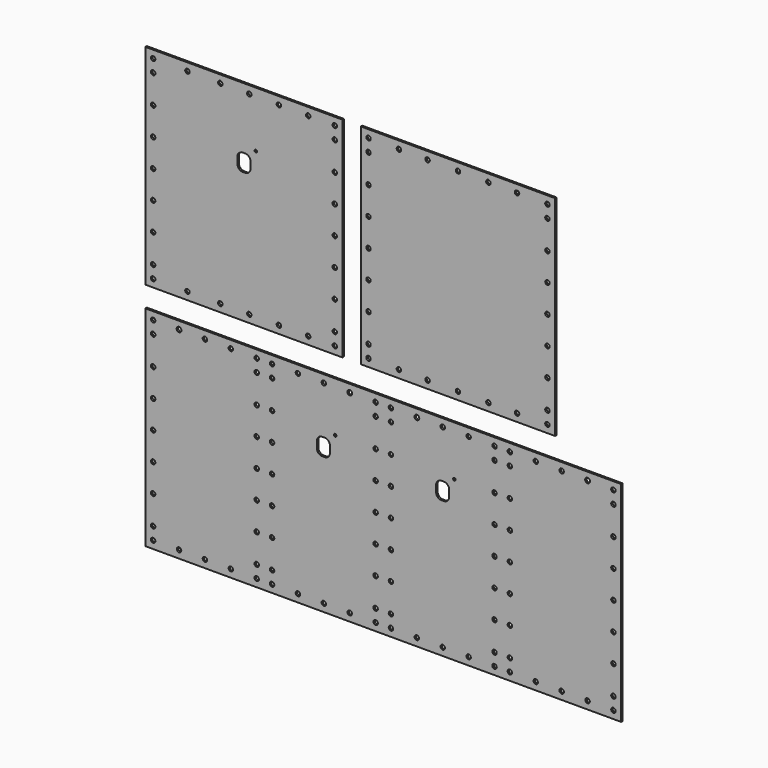
from build123d import *

# Parameters (mm, degrees)
F0_W     = 55.9308
F0_H     = 59.436
F0_R     = 0.6346933747
F0_R_2   = 0.6340066136
F0_R_3   = 0.6346542533
F0_R_4   = 0.6409040832
F0_R_5   = 0.6313502178
F0_R_6   = 0.6353923968
F0_R_7   = 0.6362020178
F0_R_8   = 0.6341762199
F0_R_9   = 0.6400206309
F0_R_10  = 0.6301156211
F0_W_2   = 3.7084
F0_H_2   = 4.8688254319
F0_R_11  = 0.3654620735
F1_DEPTH = 0.508
F0_W_3   = 55.1616173283
F0_R_12  = 0.637396124
F0_R_13  = 0.64076147
F0_R_14  = 0.6317096754
F0_W_4   = 33.7590776429
F0_R_15  = 0.634841213
F0_R_16  = 0.6334235986
F0_R_17  = 0.6322398512
F0_R_18  = 0.6856754437
F0_R_19  = 0.6353259381
F0_R_20  = 0.633153781
F2_R     = 1.524
F2_2_R   = 1.524


# Not quite as in the source:
# - two fillets or chamfers of one size are made in one step
# - a feature names something its author has since deleted; it is built from what else it names


with BuildPart() as f1:
    # F0 (on Front) → F1 (new body)
    with BuildSketch(Plane.XZ):
        Rectangle(F0_W, F0_H)
        with Locations((-25.786973536, -27.529258281)):
            Circle(F0_R, mode=Mode.SUBTRACT)
        with Locations((-16.0492006689, -27.529258281)):
            Circle(F0_R_2, mode=Mode.SUBTRACT)
        with Locations((-25.786973536, -23.9813886583)):
            Circle(F0_R_3, mode=Mode.SUBTRACT)
        with Locations((-6.7217010073, -27.529258281)):
            Circle(F0_R_4, mode=Mode.SUBTRACT)
        with Locations((1.5105993953, -27.529258281)):
            Circle(F0_R_5, mode=Mode.SUBTRACT)
        with Locations((-25.786973536, -15.8626604825)):
            Circle(F0_R_6, mode=Mode.SUBTRACT)
        with Locations((-25.786973536, -7.9313302413)):
            Circle(F0_R_7, mode=Mode.SUBTRACT)
        with Locations((9.9152876064, -27.529258281)):
            Circle(F0_R_8, mode=Mode.SUBTRACT)
        with Locations((18.2363782078, -27.529258281)):
            Circle(F0_R_9, mode=Mode.SUBTRACT)
        with Locations((25.786973536, -27.529258281)):
            Circle(F0_R, mode=Mode.SUBTRACT)
        with Locations((25.786973536, -23.9813886583)):
            Circle(F0_R_3, mode=Mode.SUBTRACT)
        with Locations((25.786973536, -15.8626604825)):
            Circle(F0_R_6, mode=Mode.SUBTRACT)
        with Locations((25.786973536, -7.9313302413)):
            Circle(F0_R_7, mode=Mode.SUBTRACT)
        with Locations((-25.786973536, 0)):
            Circle(F0_R_10, mode=Mode.SUBTRACT)
        with Locations((-25.786973536, 7.9313302413)):
            Circle(F0_R_7, mode=Mode.SUBTRACT)
        with Locations((0, 9.8690085579)):
            Rectangle(F0_W_2, F0_H_2, mode=Mode.SUBTRACT)
        with Locations((3.3375578932, 13.8644073159)):
            Circle(F0_R_11, mode=Mode.SUBTRACT)
        with Locations((-25.786973536, 15.8626604825)):
            Circle(F0_R_6, mode=Mode.SUBTRACT)
        with Locations((-25.786973536, 23.9813886583)):
            Circle(F0_R_3, mode=Mode.SUBTRACT)
        with Locations((-25.786973536, 27.529258281)):
            Circle(F0_R, mode=Mode.SUBTRACT)
        with Locations((-16.0492006689, 27.529258281)):
            Circle(F0_R_2, mode=Mode.SUBTRACT)
        with Locations((-6.7217010073, 27.529258281)):
            Circle(F0_R_4, mode=Mode.SUBTRACT)
        with Locations((1.5105993953, 27.529258281)):
            Circle(F0_R_5, mode=Mode.SUBTRACT)
        with Locations((25.786973536, 0)):
            Circle(F0_R_10, mode=Mode.SUBTRACT)
        with Locations((25.786973536, 7.9313302413)):
            Circle(F0_R_7, mode=Mode.SUBTRACT)
        with Locations((9.9152876064, 27.529258281)):
            Circle(F0_R_8, mode=Mode.SUBTRACT)
        with Locations((18.2363782078, 27.529258281)):
            Circle(F0_R_9, mode=Mode.SUBTRACT)
        with Locations((25.786973536, 15.8626604825)):
            Circle(F0_R_6, mode=Mode.SUBTRACT)
        with Locations((25.786973536, 23.9813886583)):
            Circle(F0_R_3, mode=Mode.SUBTRACT)
        with Locations((25.786973536, 27.529258281)):
            Circle(F0_R, mode=Mode.SUBTRACT)
    extrude(amount=F1_DEPTH)

    # F2
    f2_edges = [f1.edges().sort_by_distance(p)[0] for p in [
        (-1.8542, -0.254, 12.303421),
        (-1.8542, -0.254, 7.434596),
        (1.8542, -0.254, 12.303421),
        (1.8542, -0.254, 7.434596),
    ]]
    fillet(f2_edges, radius=F2_R)


with BuildPart() as f1b:
    # F0 (on Front) → F1, piece 2 (new body)
    with BuildSketch(Plane.XZ):
        with Locations((60.7584604971, 0)):
            Rectangle(F0_W_3, F0_H)
        with Locations((35.3560782969, -27.529258281)):
            Circle(F0_R, mode=Mode.SUBTRACT)
        with Locations((35.3560782969, -23.9813886583)):
            Circle(F0_R_3, mode=Mode.SUBTRACT)
        with Locations((35.3560782969, -15.8626604825)):
            Circle(F0_R_6, mode=Mode.SUBTRACT)
        with Locations((35.3560782969, -7.9313302413)):
            Circle(F0_R_7, mode=Mode.SUBTRACT)
        with Locations((35.3560782969, 0)):
            Circle(F0_R_10, mode=Mode.SUBTRACT)
        with Locations((35.3560782969, 7.9313302413)):
            Circle(F0_R_7, mode=Mode.SUBTRACT)
        with Locations((35.3560782969, 15.8626604825)):
            Circle(F0_R_6, mode=Mode.SUBTRACT)
        with Locations((35.3560782969, 23.9813886583)):
            Circle(F0_R_3, mode=Mode.SUBTRACT)
        with Locations((35.3560782969, 27.529258281)):
            Circle(F0_R, mode=Mode.SUBTRACT)
        with Locations((43.9898818731, -27.529258281)):
            Circle(F0_R_12, mode=Mode.SUBTRACT)
        with Locations((52.1195158362, -27.529258281)):
            Circle(F0_R_13, mode=Mode.SUBTRACT)
        with Locations((60.7584604971, -27.529258281)):
            Circle(F0_R_14, mode=Mode.SUBTRACT)
        with Locations((69.3974051579, -27.529258281)):
            Circle(F0_R_13, mode=Mode.SUBTRACT)
        with Locations((77.527039121, -27.529258281)):
            Circle(F0_R_12, mode=Mode.SUBTRACT)
        with Locations((86.1608426972, -27.529258281)):
            Circle(F0_R, mode=Mode.SUBTRACT)
        with Locations((86.1608426972, -23.9813886583)):
            Circle(F0_R_3, mode=Mode.SUBTRACT)
        with Locations((86.1608426972, -15.8626604825)):
            Circle(F0_R_6, mode=Mode.SUBTRACT)
        with Locations((86.1608426972, -7.9313302413)):
            Circle(F0_R_7, mode=Mode.SUBTRACT)
        with Locations((43.9898818731, 27.529258281)):
            Circle(F0_R_12, mode=Mode.SUBTRACT)
        with Locations((52.1195158362, 27.529258281)):
            Circle(F0_R_13, mode=Mode.SUBTRACT)
        with Locations((60.7584604971, 27.529258281)):
            Circle(F0_R_14, mode=Mode.SUBTRACT)
        with Locations((69.3974051579, 27.529258281)):
            Circle(F0_R_13, mode=Mode.SUBTRACT)
        with Locations((86.1608426972, 0)):
            Circle(F0_R_10, mode=Mode.SUBTRACT)
        with Locations((86.1608426972, 7.9313302413)):
            Circle(F0_R_7, mode=Mode.SUBTRACT)
        with Locations((86.1608426972, 15.8626604825)):
            Circle(F0_R_6, mode=Mode.SUBTRACT)
        with Locations((77.527039121, 27.529258281)):
            Circle(F0_R_12, mode=Mode.SUBTRACT)
        with Locations((86.1608426972, 23.9813886583)):
            Circle(F0_R_3, mode=Mode.SUBTRACT)
        with Locations((86.1608426972, 27.529258281)):
            Circle(F0_R, mode=Mode.SUBTRACT)
    extrude(amount=F1_DEPTH)


with BuildPart() as f1c:
    # F0 (on Front) → F1, piece 3 (new body)
    with BuildSketch(Plane.XZ):
        with Locations((-11.0858611785, -65.3589367867)):
            Rectangle(F0_W_4, F0_H)
        with Locations((-25.786973536, -92.8881950676)):
            Circle(F0_R, mode=Mode.SUBTRACT)
        with Locations((-25.786973536, -89.3403254449)):
            Circle(F0_R_3, mode=Mode.SUBTRACT)
        with Locations((-18.4364173573, -92.8881950676)):
            Circle(F0_R_15, mode=Mode.SUBTRACT)
        with Locations((-25.786973536, -81.2215972692)):
            Circle(F0_R_6, mode=Mode.SUBTRACT)
        with Locations((-11.0858611785, -92.8881950676)):
            Circle(F0_R_16, mode=Mode.SUBTRACT)
        with Locations((-3.7353049998, -92.8881950676)):
            Circle(F0_R_17, mode=Mode.SUBTRACT)
        with Locations((3.615251179, -92.8881950676)):
            Circle(F0_R, mode=Mode.SUBTRACT)
        with Locations((3.615251179, -89.3403254449)):
            Circle(F0_R_3, mode=Mode.SUBTRACT)
        with Locations((3.615251179, -81.2215972692)):
            Circle(F0_R_6, mode=Mode.SUBTRACT)
        with Locations((-25.786973536, -73.2902670279)):
            Circle(F0_R_7, mode=Mode.SUBTRACT)
        with Locations((-25.786973536, -65.3589367867)):
            Circle(F0_R_10, mode=Mode.SUBTRACT)
        with Locations((3.615251179, -73.2902670279)):
            Circle(F0_R_7, mode=Mode.SUBTRACT)
        with Locations((3.615251179, -65.3589367867)):
            Circle(F0_R_10, mode=Mode.SUBTRACT)
        with Locations((-25.786973536, -57.4276065454)):
            Circle(F0_R_7, mode=Mode.SUBTRACT)
        with Locations((-25.786973536, -49.4962763041)):
            Circle(F0_R_6, mode=Mode.SUBTRACT)
        with Locations((3.615251179, -57.4276065454)):
            Circle(F0_R_7, mode=Mode.SUBTRACT)
        with Locations((3.615251179, -49.4962763041)):
            Circle(F0_R_6, mode=Mode.SUBTRACT)
        with Locations((-25.786973536, -41.3775481284)):
            Circle(F0_R_3, mode=Mode.SUBTRACT)
        with Locations((-25.786973536, -37.8296785057)):
            Circle(F0_R, mode=Mode.SUBTRACT)
        with Locations((-18.4364173573, -37.8296785057)):
            Circle(F0_R_18, mode=Mode.SUBTRACT)
        with Locations((3.615251179, -41.3775481284)):
            Circle(F0_R_3, mode=Mode.SUBTRACT)
        with Locations((-11.0858611785, -37.8296785057)):
            Circle(F0_R_19, mode=Mode.SUBTRACT)
        with Locations((-3.7353049998, -37.8296785057)):
            Circle(F0_R_20, mode=Mode.SUBTRACT)
        with Locations((3.615251179, -37.8296785057)):
            Circle(F0_R, mode=Mode.SUBTRACT)
        with Locations((22.6732164644, -65.3589367867)):
            Rectangle(F0_W_4, F0_H)
        with Locations((7.9721041069, -92.8881950676)):
            Circle(F0_R, mode=Mode.SUBTRACT)
        with Locations((7.9721041069, -89.3403254449)):
            Circle(F0_R_3, mode=Mode.SUBTRACT)
        with Locations((15.3226602857, -92.8881950676)):
            Circle(F0_R_17, mode=Mode.SUBTRACT)
        with Locations((7.9721041069, -81.2215972692)):
            Circle(F0_R_6, mode=Mode.SUBTRACT)
        with Locations((22.6732164644, -92.8881950676)):
            Circle(F0_R_16, mode=Mode.SUBTRACT)
        with Locations((30.0237726432, -92.8881950676)):
            Circle(F0_R_15, mode=Mode.SUBTRACT)
        with Locations((37.3743288219, -92.8881950676)):
            Circle(F0_R, mode=Mode.SUBTRACT)
        with Locations((37.3743288219, -89.3403254449)):
            Circle(F0_R_3, mode=Mode.SUBTRACT)
        with Locations((37.3743288219, -81.2215972692)):
            Circle(F0_R_6, mode=Mode.SUBTRACT)
        with Locations((7.9721041069, -73.2902670279)):
            Circle(F0_R_7, mode=Mode.SUBTRACT)
        with Locations((7.9721041069, -65.3589367867)):
            Circle(F0_R_10, mode=Mode.SUBTRACT)
        with Locations((37.3743288219, -73.2902670279)):
            Circle(F0_R_7, mode=Mode.SUBTRACT)
        with Locations((37.3743288219, -65.3589367867)):
            Circle(F0_R_10, mode=Mode.SUBTRACT)
        with Locations((7.9721041069, -57.4276065454)):
            Circle(F0_R_7, mode=Mode.SUBTRACT)
        with Locations((7.9721041069, -49.4962763041)):
            Circle(F0_R_6, mode=Mode.SUBTRACT)
        with Locations((22.5496747531, -53.8332623895)):
            Rectangle(F0_W_2, F0_H_2, mode=Mode.SUBTRACT)
        with Locations((37.3743288219, -57.4276065454)):
            Circle(F0_R_7, mode=Mode.SUBTRACT)
        with Locations((25.8872326463, -49.8378636315)):
            Circle(F0_R_11, mode=Mode.SUBTRACT)
        with Locations((37.3743288219, -49.4962763041)):
            Circle(F0_R_6, mode=Mode.SUBTRACT)
        with Locations((7.9721041069, -41.3775481284)):
            Circle(F0_R_3, mode=Mode.SUBTRACT)
        with Locations((7.9721041069, -37.8296785057)):
            Circle(F0_R, mode=Mode.SUBTRACT)
        with Locations((15.3226602857, -37.8296785057)):
            Circle(F0_R_20, mode=Mode.SUBTRACT)
        with Locations((37.3743288219, -41.3775481284)):
            Circle(F0_R_3, mode=Mode.SUBTRACT)
        with Locations((22.6732164644, -37.8296785057)):
            Circle(F0_R_19, mode=Mode.SUBTRACT)
        with Locations((30.0237726432, -37.8296785057)):
            Circle(F0_R_18, mode=Mode.SUBTRACT)
        with Locations((37.3743288219, -37.8296785057)):
            Circle(F0_R, mode=Mode.SUBTRACT)
        with Locations((56.4322941074, -65.3589367867)):
            Rectangle(F0_W_4, F0_H)
        with Locations((41.7311817499, -92.8881950676)):
            Circle(F0_R, mode=Mode.SUBTRACT)
        with Locations((41.7311817499, -89.3403254449)):
            Circle(F0_R_3, mode=Mode.SUBTRACT)
        with Locations((49.0817379286, -92.8881950676)):
            Circle(F0_R_15, mode=Mode.SUBTRACT)
        with Locations((41.7311817499, -81.2215972692)):
            Circle(F0_R_6, mode=Mode.SUBTRACT)
        with Locations((56.4322941074, -92.8881950676)):
            Circle(F0_R_16, mode=Mode.SUBTRACT)
        with Locations((63.7828502861, -92.8881950676)):
            Circle(F0_R_17, mode=Mode.SUBTRACT)
        with Locations((71.1334064648, -92.8881950676)):
            Circle(F0_R, mode=Mode.SUBTRACT)
        with Locations((71.1334064648, -89.3403254449)):
            Circle(F0_R_3, mode=Mode.SUBTRACT)
        with Locations((71.1334064648, -81.2215972692)):
            Circle(F0_R_6, mode=Mode.SUBTRACT)
        with Locations((41.7311817499, -73.2902670279)):
            Circle(F0_R_7, mode=Mode.SUBTRACT)
        with Locations((41.7311817499, -65.3589367867)):
            Circle(F0_R_10, mode=Mode.SUBTRACT)
        with Locations((71.1334064648, -73.2902670279)):
            Circle(F0_R_7, mode=Mode.SUBTRACT)
        with Locations((71.1334064648, -65.3589367867)):
            Circle(F0_R_10, mode=Mode.SUBTRACT)
        with Locations((41.7311817499, -57.4276065454)):
            Circle(F0_R_7, mode=Mode.SUBTRACT)
        with Locations((41.7311817499, -49.4962763041)):
            Circle(F0_R_6, mode=Mode.SUBTRACT)
        with Locations((56.408532802, -53.8214271422)):
            Rectangle(F0_W_2, F0_H_2, mode=Mode.SUBTRACT)
        with Locations((71.1334064648, -57.4276065454)):
            Circle(F0_R_7, mode=Mode.SUBTRACT)
        with Locations((59.7460906953, -49.8260283843)):
            Circle(F0_R_11, mode=Mode.SUBTRACT)
        with Locations((71.1334064648, -49.4962763041)):
            Circle(F0_R_6, mode=Mode.SUBTRACT)
        with Locations((41.7311817499, -41.3775481284)):
            Circle(F0_R_3, mode=Mode.SUBTRACT)
        with Locations((41.7311817499, -37.8296785057)):
            Circle(F0_R, mode=Mode.SUBTRACT)
        with Locations((49.0817379286, -37.8296785057)):
            Circle(F0_R_18, mode=Mode.SUBTRACT)
        with Locations((71.1334064648, -41.3775481284)):
            Circle(F0_R_3, mode=Mode.SUBTRACT)
        with Locations((56.4322941074, -37.8296785057)):
            Circle(F0_R_19, mode=Mode.SUBTRACT)
        with Locations((63.7828502861, -37.8296785057)):
            Circle(F0_R_20, mode=Mode.SUBTRACT)
        with Locations((71.1334064648, -37.8296785057)):
            Circle(F0_R, mode=Mode.SUBTRACT)
        with Locations((90.1913717503, -65.3589367867)):
            Rectangle(F0_W_4, F0_H)
        with Locations((75.4902593928, -92.8881950676)):
            Circle(F0_R, mode=Mode.SUBTRACT)
        with Locations((75.4902593928, -89.3403254449)):
            Circle(F0_R_3, mode=Mode.SUBTRACT)
        with Locations((82.8408155716, -92.8881950676)):
            Circle(F0_R_17, mode=Mode.SUBTRACT)
        with Locations((75.4902593928, -81.2215972692)):
            Circle(F0_R_6, mode=Mode.SUBTRACT)
        with Locations((90.1913717503, -92.8881950676)):
            Circle(F0_R_16, mode=Mode.SUBTRACT)
        with Locations((97.541927929, -92.8881950676)):
            Circle(F0_R_15, mode=Mode.SUBTRACT)
        with Locations((104.8924841078, -92.8881950676)):
            Circle(F0_R, mode=Mode.SUBTRACT)
        with Locations((104.8924841078, -89.3403254449)):
            Circle(F0_R_3, mode=Mode.SUBTRACT)
        with Locations((104.8924841078, -81.2215972692)):
            Circle(F0_R_6, mode=Mode.SUBTRACT)
        with Locations((75.4902593928, -73.2902670279)):
            Circle(F0_R_7, mode=Mode.SUBTRACT)
        with Locations((75.4902593928, -65.3589367867)):
            Circle(F0_R_10, mode=Mode.SUBTRACT)
        with Locations((104.8924841078, -73.2902670279)):
            Circle(F0_R_7, mode=Mode.SUBTRACT)
        with Locations((104.8924841078, -65.3589367867)):
            Circle(F0_R_10, mode=Mode.SUBTRACT)
        with Locations((75.4902593928, -57.4276065454)):
            Circle(F0_R_7, mode=Mode.SUBTRACT)
        with Locations((75.4902593928, -49.4962763041)):
            Circle(F0_R_6, mode=Mode.SUBTRACT)
        with Locations((104.8924841078, -57.4276065454)):
            Circle(F0_R_7, mode=Mode.SUBTRACT)
        with Locations((104.8924841078, -49.4962763041)):
            Circle(F0_R_6, mode=Mode.SUBTRACT)
        with Locations((75.4902593928, -41.3775481284)):
            Circle(F0_R_3, mode=Mode.SUBTRACT)
        with Locations((75.4902593928, -37.8296785057)):
            Circle(F0_R, mode=Mode.SUBTRACT)
        with Locations((82.8408155716, -37.8296785057)):
            Circle(F0_R_20, mode=Mode.SUBTRACT)
        with Locations((104.8924841078, -41.3775481284)):
            Circle(F0_R_3, mode=Mode.SUBTRACT)
        with Locations((90.1913717503, -37.8296785057)):
            Circle(F0_R_19, mode=Mode.SUBTRACT)
        with Locations((97.541927929, -37.8296785057)):
            Circle(F0_R_18, mode=Mode.SUBTRACT)
        with Locations((104.8924841078, -37.8296785057)):
            Circle(F0_R, mode=Mode.SUBTRACT)
    extrude(amount=F1_DEPTH)

    # F2#2
    f2_2_edges = [f1c.edges().sort_by_distance(p)[0] for p in [
        (20.695475, -0.254, -51.39885),
        (24.403875, -0.254, -51.39885),
        (24.403875, -0.254, -56.267675),
        (20.695475, -0.254, -56.267675),
        (54.554333, -0.254, -51.387014),
        (58.262733, -0.254, -51.387014),
        (58.262733, -0.254, -56.25584),
        (54.554333, -0.254, -56.25584),
    ]]
    fillet(f2_2_edges, radius=F2_2_R)


solid = Compound([f1.part, f1b.part, f1c.part])
